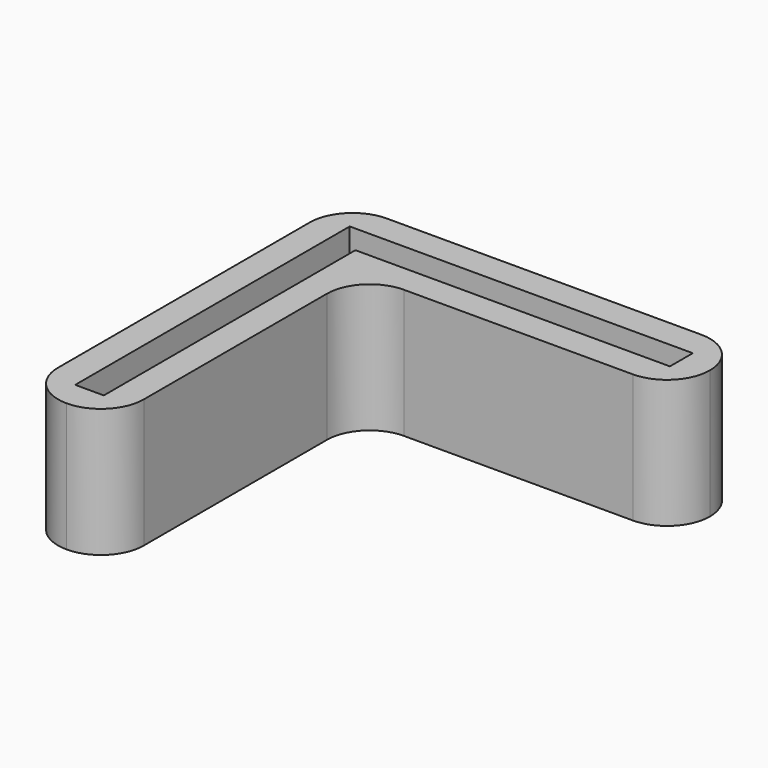
from build123d import *

# Parameters (mm, degrees)
F1_DEPTH = 2
F2_DEPTH = 7
F3_R     = 2.99999


# Not quite as in the source:
# - a fillet or chamfer is up to 0.001 mm smaller than in the source, because OpenCascade refuses the exact size


with BuildPart() as f1:
    # F0 (on Top) → F1 (new body)
    with BuildSketch(Plane.XY):
        Polygon((15.7818826017, 10.0030450644), (-10.2181173983, 10.0030450644), (-10.2181173983, -15.9969549356), (-8.2181173983, -15.9969549356), (-8.2181173983, 8.0030450644), (15.7818826017, 8.0030450644), align=None)
        Polygon((15.7818826017, 6.0030450644), (15.7818826017, 8.0030450644), (-8.2181173983, 8.0030450644), (-8.2181173983, -15.9969549356), (-6.2181173983, -15.9969549356), (-6.2181173983, 6.0030450644), align=None)
        Polygon((15.7818826017, 4.0030450644), (15.7818826017, 6.0030450644), (-6.2181173983, 6.0030450644), (-6.2181173983, -15.9969549356), (-4.2181173983, -15.9969549356), (-4.2181173983, 4.0030450644), align=None)
        Polygon((17.7818826017, 10.0030450644), (15.7818826017, 10.0030450644), (15.7818826017, 8.0030450644), (15.7818826017, 6.0030450644), (15.7818826017, 4.0030450644), (17.7818826017, 4.0030450644), align=None)
        Polygon((-8.2181173983, -15.9969549356), (-10.2181173983, -15.9969549356), (-10.2181173983, -17.9969549356), (-4.2181173983, -17.9969549356), (-4.2181173983, -15.9969549356), (-6.2181173983, -15.9969549356), align=None)
    extrude(amount=-F1_DEPTH)

    # F0 (on Top) → F2 (join)
    with BuildSketch(Plane.XY):
        Polygon((15.7818826017, 10.0030450644), (-10.2181173983, 10.0030450644), (-10.2181173983, -15.9969549356), (-8.2181173983, -15.9969549356), (-8.2181173983, 8.0030450644), (15.7818826017, 8.0030450644), align=None)
        Polygon((15.7818826017, 4.0030450644), (15.7818826017, 6.0030450644), (-6.2181173983, 6.0030450644), (-6.2181173983, -15.9969549356), (-4.2181173983, -15.9969549356), (-4.2181173983, 4.0030450644), align=None)
        Polygon((17.7818826017, 10.0030450644), (15.7818826017, 10.0030450644), (15.7818826017, 8.0030450644), (15.7818826017, 6.0030450644), (15.7818826017, 4.0030450644), (17.7818826017, 4.0030450644), align=None)
        Polygon((-8.2181173983, -15.9969549356), (-10.2181173983, -15.9969549356), (-10.2181173983, -17.9969549356), (-4.2181173983, -17.9969549356), (-4.2181173983, -15.9969549356), (-6.2181173983, -15.9969549356), align=None)
    extrude(amount=F2_DEPTH)

    # F3 (radius 3 in the source; OpenCascade refuses exactly that, so slightly less here)
    f3_edges = [f1.edges().sort_by_distance(p)[0] for p in [
        (-4.218117, 4.003045, 2.5),
        (-10.218117, 10.003045, 2.5),
        (-10.218117, -17.996955, 2.5),
        (-4.218117, -17.996955, 2.5),
        (17.781883, 4.003045, 2.5),
        (17.781883, 10.003045, 2.5),
    ]]
    fillet(f3_edges, radius=F3_R)


solid = f1.part
